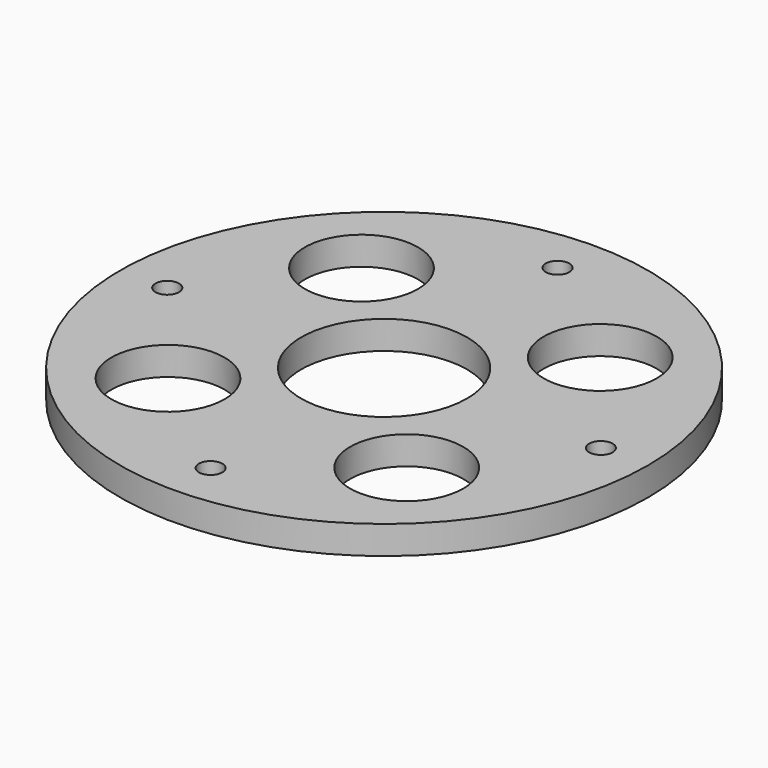
from build123d import *

# Parameters (mm, degrees)
F0_R     = 88.9
F0_R_2   = 19.05
F0_R_3   = 3.96875
F0_R_4   = 27.94
F1_DEPTH = 9.525


# Not quite as in the source:
# - a length typed as a fraction of an inch, garbled in the dataset ("3 / 203.2 mm" for 3/8 in), is restored


with BuildPart() as f1:
    # F0 (on Top) → F1 (new body)
    with BuildSketch(Plane.XY):
        Circle(F0_R)
        with Locations((-40.6679487148, -40.1527140717)):
            Circle(F0_R_2, mode=Mode.SUBTRACT)
        with Locations((0, -73.025)):
            Circle(F0_R_3, mode=Mode.SUBTRACT)
        with Locations((40.1527140717, -40.6679487148)):
            Circle(F0_R_2, mode=Mode.SUBTRACT)
        with Locations((-73.025, 0)):
            Circle(F0_R_3, mode=Mode.SUBTRACT)
        with Locations((-40.1527140717, 40.6679487148)):
            Circle(F0_R_2, mode=Mode.SUBTRACT)
        Circle(F0_R_4, mode=Mode.SUBTRACT)
        with Locations((40.6679487148, 40.1527140717)):
            Circle(F0_R_2, mode=Mode.SUBTRACT)
        with Locations((73.025, 0)):
            Circle(F0_R_3, mode=Mode.SUBTRACT)
        with Locations((0, 73.025)):
            Circle(F0_R_3, mode=Mode.SUBTRACT)
    extrude(amount=F1_DEPTH)


solid = f1.part
